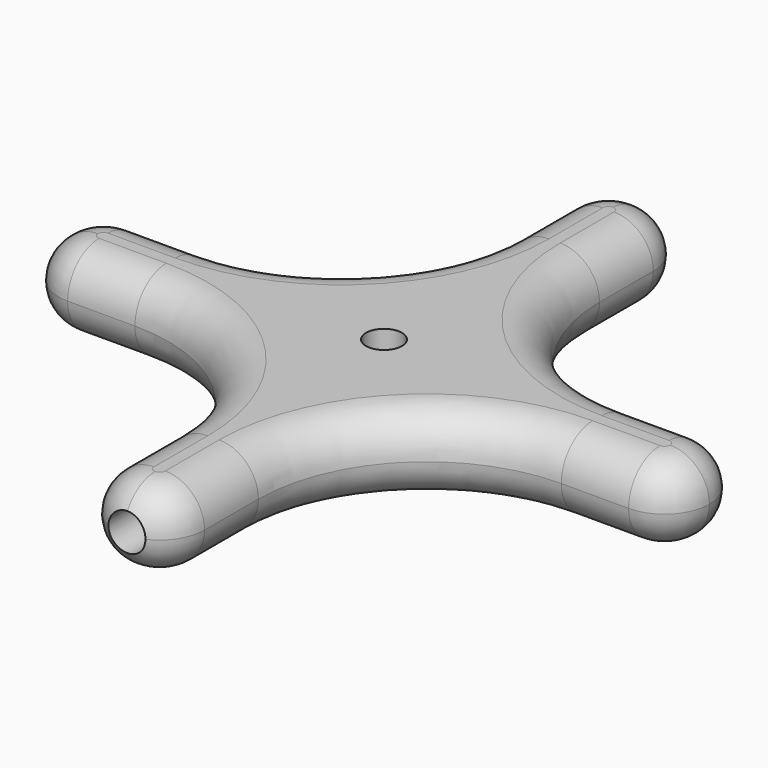
from build123d import *

# Parameters (mm, degrees)
F0_R     = 3.2
F1_DEPTH = 14
F2_R     = 7
F3_R     = 6.99999
F5_START = 5
F4_R     = 3.3
F5_DEPTH = 60
F7_START = -5
F6_R     = 3.3
F7_DEPTH = 60


# Not quite as in the source:
# - a fillet or chamfer is up to 0.001 mm smaller than in the source, because OpenCascade refuses the exact size


with BuildPart() as f1:
    # F0 (on Top) → F1 (new body)
    with BuildSketch(Plane.XY):
        with BuildLine():
            ThreePointArc((0, 58), (-5.6568542495, 55.6568542495), (-8, 50))
            Line((-8, 50), (-8, 38))
            ThreePointArc((-8, 38), (-16.7867965644, 16.7867965644), (-38, 8))
            Line((-38, 8), (-50, 8))
            ThreePointArc((-50, 8), (-55.6568542495, 5.6568542495), (-58, 0))
            ThreePointArc((-58, 0), (-55.6568542495, -5.6568542495), (-50, -8))
            Line((-50, -8), (-38, -8))
            ThreePointArc((-38, -8), (-16.7867965644, -16.7867965644), (-8, -38))
            Line((-8, -38), (-8, -50))
            ThreePointArc((-8, -50), (-5.6568542495, -55.6568542495), (0, -58))
            ThreePointArc((0, -58), (5.6568542495, -55.6568542495), (8, -50))
            Line((8, -50), (8, -38))
            ThreePointArc((8, -38), (16.7867965644, -16.7867965644), (38, -8))
            Line((38, -8), (50, -8))
            ThreePointArc((50, -8), (55.6568542495, -5.6568542495), (58, 0))
            ThreePointArc((58, 0), (55.6568542495, 5.6568542495), (50, 8))
            Line((50, 8), (38, 8))
            ThreePointArc((38, 8), (16.7867965644, 16.7867965644), (8, 38))
            Line((8, 38), (8, 50))
            ThreePointArc((8, 50), (5.6568542495, 55.6568542495), (0, 58))
        make_face()
        Circle(F0_R, mode=Mode.SUBTRACT)
    extrude(amount=F1_DEPTH)

    # F2
    f2_edges = [f1.edges().sort_by_distance(p)[0] for p in [
        (-16.786797, 16.786797, 14),
    ]]
    fillet(f2_edges, radius=F2_R)

    # F3 (radius 7 in the source; OpenCascade refuses exactly that, so slightly less here)
    f3_edges = [f1.edges().sort_by_distance(p)[0] for p in [
        (16.786797, 16.786797, 0),
    ]]
    fillet(f3_edges, radius=F3_R)

    # F4 (on Front) → F5 (cut)
    with BuildSketch(Plane.XZ.offset(F5_START)):
        with Locations((0, 7)):
            Circle(F4_R)
    extrude(amount=F5_DEPTH, mode=Mode.SUBTRACT)

    # F6 (on Right) → F7 (cut)
    with BuildSketch(Plane.YZ.offset(F7_START)):
        with Locations((0, 7)):
            Circle(F6_R)
    extrude(amount=-F7_DEPTH, mode=Mode.SUBTRACT)


solid = f1.part
